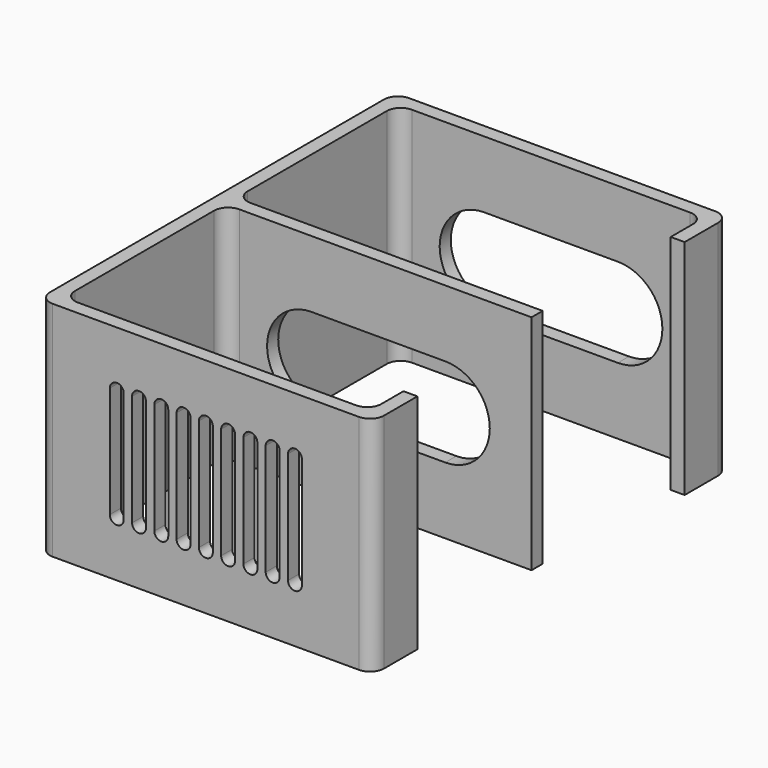
from build123d import *

# Parameters (mm, degrees)
F2_W          = 55
F2_H          = 2.5
F4_DEPTH      = 40
F6_DEPTH      = 2.501
F6_DEPTH_BACK = 75
F8_DEPTH      = 2.501
F9_R          = 2.5


with BuildPart() as f4:
    # F2 (on Top) → F4 (new body)
    with BuildSketch(Plane.XY):
        with Locations((30, 40)):
            Rectangle(F2_W, F2_H)
        Polygon((0, 80), (0, 0), (60, 0), (60, 10), (57.5, 10), (57.5, 2.5), (2.5, 2.5), (2.5, 38.75), (2.5, 41.25), (2.5, 77.5), (57.5, 77.5), (57.5, 70), (60, 70), (60, 80), align=None)
    extrude(amount=F4_DEPTH)

    # F5 (on face) → F6 (cut, two sides)
    with BuildSketch(Plane.XZ.offset(-77.5)) as f6_sk:
        with BuildLine():
            ThreePointArc((18, 12), (23.6568542495, 14.3431457505), (26, 20))
            ThreePointArc((26, 20), (23.6568542495, 25.6568542495), (18, 28))
            ThreePointArc((18, 28), (10, 20), (18, 12))
        make_face()
        with BuildLine():
            ThreePointArc((18, 28), (23.6568542495, 25.6568542495), (26, 20))
            ThreePointArc((26, 20), (23.6568542495, 14.3431457505), (18, 12))
            Line((18, 12), (42, 12))
            ThreePointArc((42, 12), (34, 20), (42, 28))
            Line((42, 28), (18, 28))
        make_face()
        with BuildLine():
            ThreePointArc((50, 20), (47.6568542495, 25.6568542495), (42, 28))
            ThreePointArc((42, 28), (34, 20), (42, 12))
            ThreePointArc((42, 12), (47.6568542495, 14.3431457505), (50, 20))
        make_face()
    extrude(amount=-F6_DEPTH, mode=Mode.SUBTRACT)
    extrude(f6_sk.sketch, amount=F6_DEPTH_BACK, mode=Mode.SUBTRACT)

    # F7 (on face) → F8 (cut, through all)
    with BuildSketch(Plane(origin=(0, 2.5, 0), x_dir=(-1, 0, 0), z_dir=(0, 1, 0))):
        with BuildLine():
            ThreePointArc((-15.25, 30), (-14, 28.75), (-12.75, 30))
            ThreePointArc((-12.75, 30), (-14, 31.25), (-15.25, 30))
        make_face()
        with BuildLine():
            ThreePointArc((-15.25, 10), (-14, 11.25), (-12.75, 10))
            Line((-12.75, 10), (-12.75, 30))
            ThreePointArc((-12.75, 30), (-14, 28.75), (-15.25, 30))
            Line((-15.25, 30), (-15.25, 10))
        make_face()
        with BuildLine():
            ThreePointArc((-15.25, 10), (-14, 8.75), (-12.75, 10))
            ThreePointArc((-12.75, 10), (-14, 11.25), (-15.25, 10))
        make_face()
        with BuildLine():
            ThreePointArc((-19.25, 10), (-18, 8.75), (-16.75, 10))
            ThreePointArc((-16.75, 10), (-18, 11.25), (-19.25, 10))
        make_face()
        with BuildLine():
            ThreePointArc((-19.25, 10), (-18, 11.25), (-16.75, 10))
            Line((-16.75, 10), (-16.75, 30))
            ThreePointArc((-16.75, 30), (-18, 28.75), (-19.25, 30))
            Line((-19.25, 30), (-19.25, 10))
        make_face()
        with BuildLine():
            ThreePointArc((-19.25, 30), (-18, 28.75), (-16.75, 30))
            ThreePointArc((-16.75, 30), (-18, 31.25), (-19.25, 30))
        make_face()
        with BuildLine():
            ThreePointArc((-23.25, 30), (-22, 28.75), (-20.75, 30))
            ThreePointArc((-20.75, 30), (-22, 31.25), (-23.25, 30))
        make_face()
        with BuildLine():
            ThreePointArc((-23.25, 10), (-22, 11.25), (-20.75, 10))
            Line((-20.75, 10), (-20.75, 30))
            ThreePointArc((-20.75, 30), (-22, 28.75), (-23.25, 30))
            Line((-23.25, 30), (-23.25, 10))
        make_face()
        with BuildLine():
            ThreePointArc((-23.25, 10), (-22, 8.75), (-20.75, 10))
            ThreePointArc((-20.75, 10), (-22, 11.25), (-23.25, 10))
        make_face()
        with BuildLine():
            ThreePointArc((-27.25, 10), (-26, 8.75), (-24.75, 10))
            ThreePointArc((-24.75, 10), (-26, 11.25), (-27.25, 10))
        make_face()
        with BuildLine():
            ThreePointArc((-27.25, 30), (-26, 28.75), (-24.75, 30))
            ThreePointArc((-24.75, 30), (-26, 31.25), (-27.25, 30))
        make_face()
        with BuildLine():
            ThreePointArc((-31.25, 30), (-30, 28.75), (-28.75, 30))
            ThreePointArc((-28.75, 30), (-30, 31.25), (-31.25, 30))
        make_face()
        with BuildLine():
            Line((-28.75, 10), (-28.75, 30))
            ThreePointArc((-28.75, 30), (-30, 28.75), (-31.25, 30))
            Line((-31.25, 30), (-31.25, 10))
            ThreePointArc((-31.25, 10), (-30, 11.25), (-28.75, 10))
        make_face()
        with BuildLine():
            ThreePointArc((-31.25, 10), (-30, 8.75), (-28.75, 10))
            ThreePointArc((-28.75, 10), (-30, 11.25), (-31.25, 10))
        make_face()
        with BuildLine():
            ThreePointArc((-27.25, 10), (-26, 11.25), (-24.75, 10))
            Line((-24.75, 10), (-24.75, 30))
            ThreePointArc((-24.75, 30), (-26, 28.75), (-27.25, 30))
            Line((-27.25, 30), (-27.25, 10))
        make_face()
        with BuildLine():
            ThreePointArc((-32.75, 10), (-34, 11.25), (-35.25, 10))
            ThreePointArc((-35.25, 10), (-34, 8.75), (-32.75, 10))
        make_face()
        with BuildLine():
            ThreePointArc((-32.75, 30), (-34, 28.75), (-35.25, 30))
            Line((-35.25, 30), (-35.25, 10))
            ThreePointArc((-35.25, 10), (-34, 11.25), (-32.75, 10))
            Line((-32.75, 10), (-32.75, 30))
        make_face()
        with BuildLine():
            ThreePointArc((-32.75, 30), (-34, 31.25), (-35.25, 30))
            ThreePointArc((-35.25, 30), (-34, 28.75), (-32.75, 30))
        make_face()
        with BuildLine():
            ThreePointArc((-36.75, 30), (-38, 31.25), (-39.25, 30))
            ThreePointArc((-39.25, 30), (-38, 28.75), (-36.75, 30))
        make_face()
        with BuildLine():
            ThreePointArc((-36.75, 30), (-38, 28.75), (-39.25, 30))
            Line((-39.25, 30), (-39.25, 10))
            ThreePointArc((-39.25, 10), (-38, 11.25), (-36.75, 10))
            Line((-36.75, 10), (-36.75, 30))
        make_face()
        with BuildLine():
            ThreePointArc((-36.75, 10), (-38, 11.25), (-39.25, 10))
            ThreePointArc((-39.25, 10), (-38, 8.75), (-36.75, 10))
        make_face()
        with BuildLine():
            ThreePointArc((-40.75, 10), (-42, 11.25), (-43.25, 10))
            ThreePointArc((-43.25, 10), (-42, 8.75), (-40.75, 10))
        make_face()
        with BuildLine():
            ThreePointArc((-40.75, 30), (-42, 28.75), (-43.25, 30))
            Line((-43.25, 30), (-43.25, 10))
            ThreePointArc((-43.25, 10), (-42, 11.25), (-40.75, 10))
            Line((-40.75, 10), (-40.75, 30))
        make_face()
        with BuildLine():
            ThreePointArc((-40.75, 30), (-42, 31.25), (-43.25, 30))
            ThreePointArc((-43.25, 30), (-42, 28.75), (-40.75, 30))
        make_face()
        with BuildLine():
            ThreePointArc((-44.75, 30), (-46, 31.25), (-47.25, 30))
            ThreePointArc((-47.25, 30), (-46, 28.75), (-44.75, 30))
        make_face()
        with BuildLine():
            ThreePointArc((-44.75, 30), (-46, 28.75), (-47.25, 30))
            Line((-47.25, 30), (-47.25, 10))
            ThreePointArc((-47.25, 10), (-46, 11.25), (-44.75, 10))
            Line((-44.75, 10), (-44.75, 30))
        make_face()
        with BuildLine():
            ThreePointArc((-44.75, 10), (-46, 11.25), (-47.25, 10))
            ThreePointArc((-47.25, 10), (-46, 8.75), (-44.75, 10))
        make_face()
    extrude(amount=-F8_DEPTH, mode=Mode.SUBTRACT)

    # F9
    f9_edges = [f4.edges().sort_by_distance(p)[0] for p in [
        (2.5, 41.25, 20),
        (2.5, 38.75, 20),
        (2.5, 77.5, 20),
        (60, 80, 20),
        (57.5, 77.5, 20),
        (0, 80, 20),
        (2.5, 2.5, 20),
        (57.5, 2.5, 20),
        (0, 0, 20),
        (60, 0, 20),
    ]]
    fillet(f9_edges, radius=F9_R)


solid = f4.part
